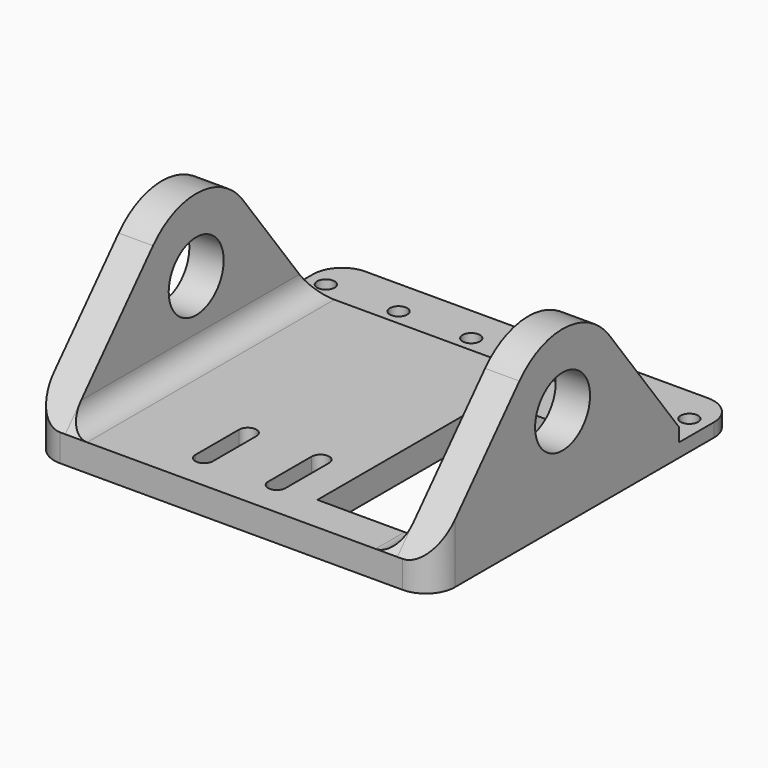
from build123d import *

# Parameters (mm, degrees)
F0_W          = 70
F0_H          = 66.675
F1_DEPTH      = 4.7625
F2_R          = 6
F3_DEPTH      = 70
F4_W          = 58
F4_H          = 53.975
F5_DEPTH      = 25.401
F6_W          = 15.875
F6_H          = 38.1
F7_DEPTH      = 4.7625
F9_DEPTH      = 25.4
F10_W         = 70
F10_H         = 12.7
F11_DEPTH     = 2.38125
F12_R         = 1.524
F13_DEPTH     = 2.38125
F14_R         = 5.08
F15_T4_DEPTH  = 53.975
F15_T10_DEPTH = 53.975
F15_T17_DEPTH = 53.975
F15_T24_DEPTH = 53.975
F15_T31_DEPTH = 53.975
F15_T38_DEPTH = 53.975
F16_R         = 5.08


# Not quite as in the source:
# - a fillet or chamfer that OpenCascade refuses, or shapes differently, is made with other operations: its cross-section is extruded or revolved along the edge and cut away or added
# - a feature of the source that left no trace in its solid (it failed there, or was rolled back) is left out


with BuildPart() as f1:
    # F0 (on Top) → F1 (new body)
    with BuildSketch(Plane.XY):
        Rectangle(F0_W, F0_H)
    extrude(amount=F1_DEPTH)

    # F2 (on face) → F3 (join, through all)
    with BuildSketch(Plane(origin=(-35, 0, 0), x_dir=(0, -1, 0), z_dir=(-1, 0, 0))):
        with BuildLine():
            ThreePointArc((-5.3975, 25.0825), (-7.2857778852, 21.4785926284), (-7.9375, 17.4625))
            Line((-7.9375, 17.4625), (-7.9375, 4.7625))
            Line((-7.9375, 4.7625), (17.4625, 4.7625))
            Line((17.4625, 4.7625), (17.4625, 17.4625))
            ThreePointArc((17.4625, 17.4625), (16.6159891988, 22.0215343072), (14.1893041237, 25.9728092784))
            ThreePointArc((14.1893041237, 25.9728092784), (4.1858227063, 30.1494004607), (-5.3975, 25.0825))
        make_face()
        with Locations((4.7625, 17.4625)):
            Circle(F2_R, mode=Mode.SUBTRACT)
        with BuildLine():
            Line((-7.9375, 4.7625), (-7.9375, 17.4625))
            ThreePointArc((-7.9375, 17.4625), (-7.2857778852, 21.4785926284), (-5.3975, 25.0825))
            Line((-5.3975, 25.0825), (-20.6375, 4.7625))
            Line((-20.6375, 4.7625), (-7.9375, 4.7625))
        make_face()
        with BuildLine():
            Line((17.4625, 17.4625), (17.4625, 4.7625))
            Line((17.4625, 4.7625), (33.3375, 4.7625))
            Line((33.3375, 4.7625), (14.1893041237, 25.9728092784))
            ThreePointArc((14.1893041237, 25.9728092784), (16.6159891988, 22.0215343072), (17.4625, 17.4625))
        make_face()
    extrude(amount=-F3_DEPTH)

    # F4 (on face) → F5 (cut, through all)
    with BuildSketch(Plane.XY.offset(4.7625)):
        with Locations((0, -6.35)):
            Rectangle(F4_W, F4_H)
    extrude(amount=F5_DEPTH, mode=Mode.SUBTRACT)

    # F6 (on face) → F7 (cut, through all)
    with BuildSketch(Plane.XY.offset(4.7625)):
        with Locations((17.8875, -7.9375)):
            Rectangle(F6_W, F6_H)
    extrude(amount=-F7_DEPTH, mode=Mode.SUBTRACT)

    # F8 (on face) → F9 (cut)
    with BuildSketch(Plane(origin=(0, 0, 0), x_dir=(1, 0, 0), z_dir=(0, 0, -1))):
        with BuildLine():
            Line((1.345, 26.9875), (1.345, 17.4625))
            ThreePointArc((1.345, 17.4625), (2.869, 15.9385), (4.393, 17.4625))
            Line((4.393, 17.4625), (4.393, 26.9875))
            ThreePointArc((4.393, 26.9875), (2.869, 28.5115), (1.345, 26.9875))
        make_face()
        with BuildLine():
            Line((-11.355, 26.9875), (-11.355, 17.4625))
            ThreePointArc((-11.355, 17.4625), (-9.831, 15.9385), (-8.307, 17.4625))
            Line((-8.307, 17.4625), (-8.307, 26.9875))
            ThreePointArc((-8.307, 26.9875), (-9.831, 28.5115), (-11.355, 26.9875))
        make_face()
    extrude(amount=-F9_DEPTH, mode=Mode.SUBTRACT)

    # F10 (on face) → F11 (cut)
    with BuildSketch(Plane.XY.offset(4.7625)):
        with Locations((0, 26.9875)):
            Rectangle(F10_W, F10_H)
    extrude(amount=-F11_DEPTH, mode=Mode.SUBTRACT)

    # F12 (on face) → F13 (cut, through all)
    with BuildSketch(Plane.XY.offset(2.38125)):
        with Locations((-31.75, 26.9875)):
            Circle(F12_R)
        with Locations((-19.05, 26.9875)):
            Circle(F12_R)
        with Locations((-6.35, 26.9875)):
            Circle(F12_R)
        with Locations((6.35, 26.9875)):
            Circle(F12_R)
        with Locations((19.05, 26.9875)):
            Circle(F12_R)
        with Locations((31.75, 26.9875)):
            Circle(F12_R)
    extrude(amount=-F13_DEPTH, mode=Mode.SUBTRACT)

    # F14
    f14_edges = [f1.edges().sort_by_distance(p)[0] for p in [
        (-35, 33.3375, 1.190625),
        (35, 33.3375, 1.190625),
    ]]
    fillet(f14_edges, radius=F14_R)

    # F15: fillet of radius 3.81 on 2 edges, made by hand


with BuildPart() as f15_tool2:
    # F15_s3 → F15_t4 (new body)
    with BuildSketch(Plane.XZ.offset(-20.6375)):
        with BuildLine():
            ThreePointArc((-25.19, 4.7625), (-27.8840768363, 5.8784231637), (-29, 8.5725))
            Line((-29, 8.5725), (-29, 4.7625))
            Line((-29, 4.7625), (-25.19, 4.7625))
        make_face()
    extrude(amount=F15_T4_DEPTH)

    split(bisect_by=Plane(origin=(0, -20.7365394835, 18.7204870337), x_dir=(1, 0, 0), z_dir=(0, 0.7422680412, -0.6701030928)), keep=Keep.TOP)

    split(bisect_by=Plane(origin=(0, 15.494, 11.6205), x_dir=(1, 0, 0), z_dir=(0, -0.8, -0.6)), keep=Keep.TOP)


with BuildPart() as f1_1:
    add(f1.part)

    # F15_t1: union F15_tool2
    add(f15_tool2.part)


with BuildPart() as f15_tool8:
    # F15_s9 → F15_t10 (new body)
    with BuildSketch(Plane.XZ.offset(33.3375)):
        with BuildLine():
            ThreePointArc((25.19, 4.7625), (27.8840768363, 5.8784231637), (29, 8.5725))
            Line((29, 8.5725), (29, 4.7625))
            Line((29, 4.7625), (25.19, 4.7625))
        make_face()
    extrude(amount=-F15_T10_DEPTH)

    split(bisect_by=Plane(origin=(0, -20.7365394835, 18.7204870337), x_dir=(1, 0, 0), z_dir=(0, 0.7422680412, -0.6701030928)), keep=Keep.TOP)

    split(bisect_by=Plane.XZ.offset(26.9875), keep=Keep.TOP)

    split(bisect_by=Plane.YZ.offset(25.825), keep=Keep.BOTTOM)


with BuildPart() as f1_2:
    add(f1_1.part)

    # F15_t7: union F15_tool8
    add(f15_tool8.part)


with BuildPart() as f15_tool15:
    # F15_s16 → F15_t17 (new body)
    with BuildSketch(Plane.XZ.offset(33.3375)):
        with BuildLine():
            ThreePointArc((25.19, 4.7625), (27.8840768363, 5.8784231637), (29, 8.5725))
            Line((29, 8.5725), (29, 4.7625))
            Line((29, 4.7625), (25.19, 4.7625))
        make_face()
    extrude(amount=-F15_T17_DEPTH)

    split(bisect_by=Plane(origin=(0, -20.7365394835, 18.7204870337), x_dir=(1, 0, 0), z_dir=(0, 0.7422680412, -0.6701030928)), keep=Keep.TOP)

    split(bisect_by=Plane.XZ.offset(26.9875), keep=Keep.TOP)

    split(bisect_by=Plane.YZ.offset(25.825), keep=Keep.TOP)


with BuildPart() as f1_3:
    add(f1_2.part)

    # F15_t14: union F15_tool15
    add(f15_tool15.part)


with BuildPart() as f15_tool22:
    # F15_s23 → F15_t24 (new body)
    with BuildSketch(Plane.XZ.offset(33.3375)):
        with BuildLine():
            ThreePointArc((25.19, 4.7625), (27.8840768363, 5.8784231637), (29, 8.5725))
            Line((29, 8.5725), (29, 4.7625))
            Line((29, 4.7625), (25.19, 4.7625))
        make_face()
    extrude(amount=-F15_T24_DEPTH)

    split(bisect_by=Plane.XZ.offset(26.9875), keep=Keep.BOTTOM)

    split(bisect_by=Plane.YZ.offset(25.825), keep=Keep.TOP)

    split(bisect_by=Plane.XZ.offset(-11.1125), keep=Keep.TOP)


with BuildPart() as f1_4:
    add(f1_3.part)

    # F15_t21: union F15_tool22
    add(f15_tool22.part)


with BuildPart() as f15_tool29:
    # F15_s30 → F15_t31 (new body)
    with BuildSketch(Plane.XZ.offset(33.3375)):
        with BuildLine():
            ThreePointArc((25.19, 4.7625), (27.8840768363, 5.8784231637), (29, 8.5725))
            Line((29, 8.5725), (29, 4.7625))
            Line((29, 4.7625), (25.19, 4.7625))
        make_face()
    extrude(amount=-F15_T31_DEPTH)

    split(bisect_by=Plane(origin=(0, 15.494, 11.6205), x_dir=(1, 0, 0), z_dir=(0, -0.8, -0.6)), keep=Keep.TOP)

    split(bisect_by=Plane.YZ.offset(25.825), keep=Keep.BOTTOM)

    split(bisect_by=Plane.XZ.offset(-11.1125), keep=Keep.BOTTOM)


with BuildPart() as f1_5:
    add(f1_4.part)

    # F15_t28: union F15_tool29
    add(f15_tool29.part)


with BuildPart() as f15_tool36:
    # F15_s37 → F15_t38 (new body)
    with BuildSketch(Plane.XZ.offset(33.3375)):
        with BuildLine():
            ThreePointArc((25.19, 4.7625), (27.8840768363, 5.8784231637), (29, 8.5725))
            Line((29, 8.5725), (29, 4.7625))
            Line((29, 4.7625), (25.19, 4.7625))
        make_face()
    extrude(amount=-F15_T38_DEPTH)

    split(bisect_by=Plane(origin=(0, 15.494, 11.6205), x_dir=(1, 0, 0), z_dir=(0, -0.8, -0.6)), keep=Keep.TOP)

    split(bisect_by=Plane.YZ.offset(25.825), keep=Keep.TOP)

    split(bisect_by=Plane.XZ.offset(-11.1125), keep=Keep.BOTTOM)


with BuildPart() as f1_6:
    add(f1_5.part)

    # F15_t35: union F15_tool36
    add(f15_tool36.part)

    # F16
    f16_edges = [f1_6.edges().sort_by_distance(p)[0] for p in [
        (35, -33.3375, 2.38125),
        (-35, -33.3375, 2.38125),
    ]]
    fillet(f16_edges, radius=F16_R)


solid = f1_6.part
